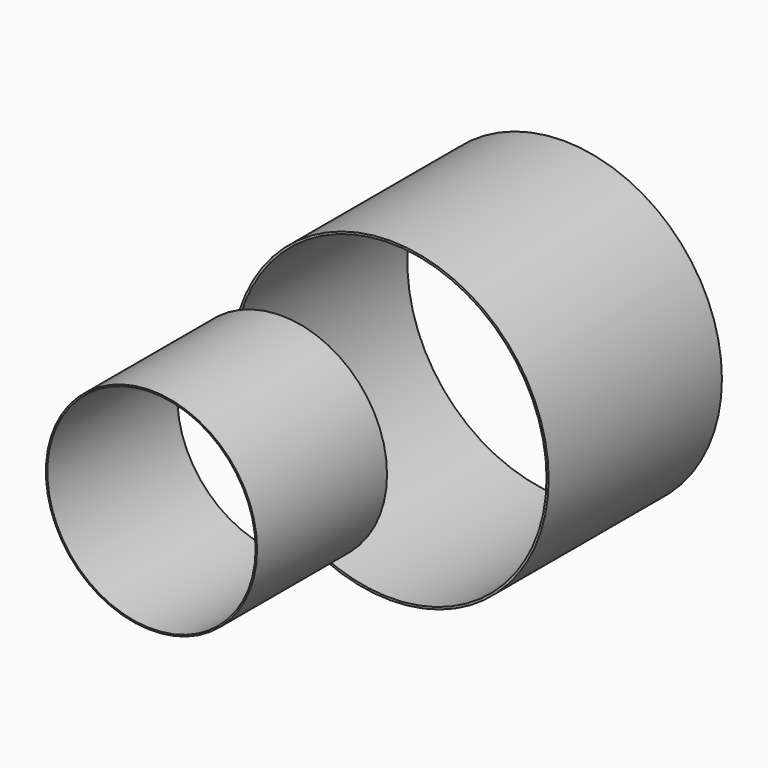
from build123d import *

# Parameters (mm, degrees)
F0_R     = 38
F0_R_2   = 37.5
F1_DEPTH = 52
F3_R     = 25.35
F3_R_2   = 25
F4_DEPTH = 39


# Not quite as in the source:
# - the program builds the solid bodies; features that only make, move or delete a surface that nothing else refers to are left out


with BuildPart() as f1:
    # F0 (on Front) → F1 (new body)
    with BuildSketch(Plane.XZ):
        Circle(F0_R)
        Circle(F0_R_2, mode=Mode.SUBTRACT)
    extrude(amount=F1_DEPTH)


with BuildPart() as f4:
    # F3 (on offset) → F4 (new body)
    with BuildSketch(Plane.XZ.offset(69.5)):
        with Locations((-12.15, 0)):
            Circle(F3_R)
        with Locations((-12.15, 0)):
            Circle(F3_R_2, mode=Mode.SUBTRACT)
    extrude(amount=F4_DEPTH)


solid = Compound([f1.part, f4.part])
